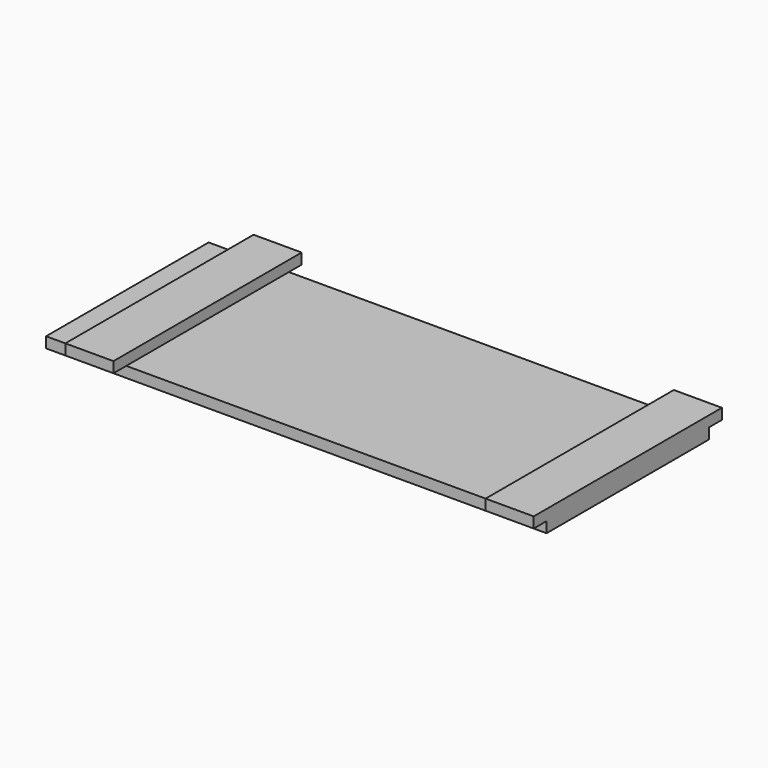
from build123d import *

# Parameters (mm, degrees)
F0_W     = 38.1
F0_H     = 241.3
F0_W_2   = 57.15
F0_W_3   = 441.96
F1_DEPTH = 12.7
F0_H_2   = 19.05
F2_DEPTH = 12.7


# Not quite as in the source:
# - a feature names something its author has since deleted; it is built from what else it names


with BuildPart() as f1:
    # F0 (on Top) → F1 (new body)
    with BuildSketch(Plane.XY):
        with Locations((-278.13, 0)):
            Rectangle(F0_W, F0_H)
        with Locations((-230.505, 0)):
            Rectangle(F0_W_2, F0_H)
        with Locations((19.05, 0)):
            Rectangle(F0_W_3, F0_H)
        with Locations((268.605, 0)):
            Rectangle(F0_W_2, F0_H)
    extrude(amount=-F1_DEPTH)

    # F0 (on Top) → F2 (join)
    with BuildSketch(Plane.XY):
        with Locations((-230.505, 130.175)):
            Rectangle(F0_W_2, F0_H_2)
        with Locations((-230.505, -130.175)):
            Rectangle(F0_W_2, F0_H_2)
        with Locations((-230.505, 0)):
            Rectangle(F0_W_2, F0_H)
        with Locations((268.605, 0)):
            Rectangle(F0_W_2, F0_H)
        with Locations((268.605, -130.175)):
            Rectangle(F0_W_2, F0_H_2)
        with Locations((268.605, 130.175)):
            Rectangle(F0_W_2, F0_H_2)
    extrude(amount=F2_DEPTH)


solid = f1.part
